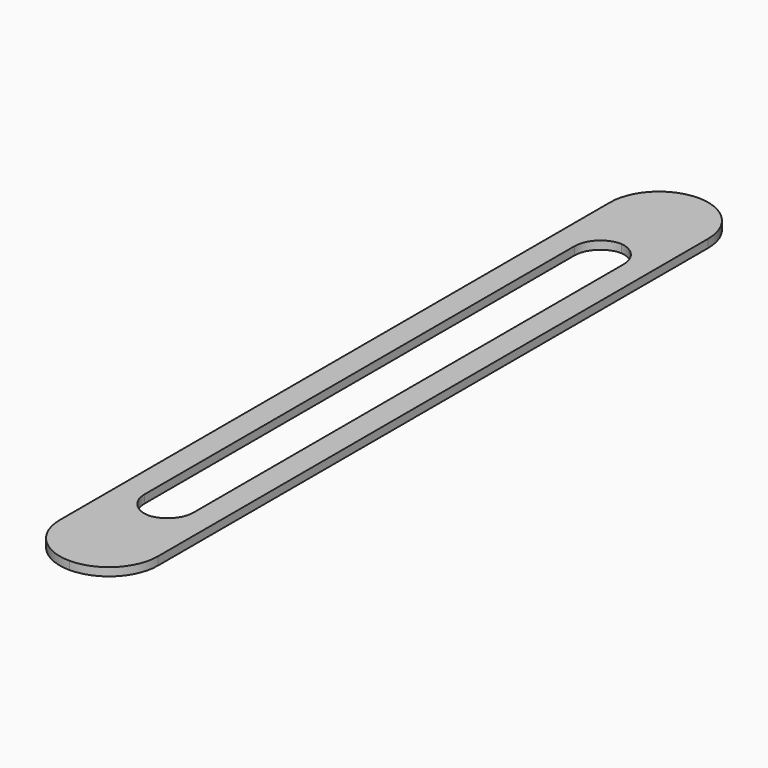
from build123d import *

# Parameters (mm, degrees)
F0_W        = 19.05
F0_H        = 152.4
F1_DEPTH    = 1.5875
F2_R        = 9.52499
F4_W        = 9.525
F4_H        = 114.3
F5_DEPTH    = 25.4
F6_T1_DEPTH = 1.5875
F7_T1_DEPTH = 1.5875


# Not quite as in the source:
# - a fillet or chamfer that OpenCascade refuses, or shapes differently, is made with other operations: its cross-section is extruded or revolved along the edge and cut away or added
# - a fillet or chamfer is up to 0.001 mm smaller than in the source, because OpenCascade refuses the exact size


with BuildPart() as f1:
    # F0 (on Top) → F1 (new body)
    with BuildSketch(Plane.XY):
        with Locations((-58.0996136427, 28.9993500233)):
            Rectangle(F0_W, F0_H)
    extrude(amount=-F1_DEPTH)

    # F2 (radius 9.525 in the source; OpenCascade refuses exactly that, so slightly less here)
    f2_edges = [f1.edges().sort_by_distance(p)[0] for p in [
        (-48.574614, -47.20065, -0.79375),
        (-67.624614, -47.20065, -0.79375),
        (-48.574614, 105.19935, -0.79375),
        (-67.624614, 105.19935, -0.79375),
    ]]
    fillet(f2_edges, radius=F2_R)

    # F4 (on offset) → F5 (cut)
    with BuildSketch(Plane.XY):
        with Locations((-58.0996136427, 28.9993500233)):
            Rectangle(F4_W, F4_H)
    extrude(amount=-F5_DEPTH, mode=Mode.SUBTRACT)

    # F6: fillet of radius 5.08 on 3 edges, made by hand

    # F6_s2 → F6_t1 (join)
    with BuildSketch(Plane.XY.offset(-1.5875)):
        with BuildLine():
            ThreePointArc((-62.8621136427, -23.0706499767), (-61.3742160911, -26.6627524252), (-57.7821136427, -28.1506499767))
            Line((-57.7821136427, -28.1506499767), (-62.8621136427, -28.1506499767))
            Line((-62.8621136427, -28.1506499767), (-62.8621136427, -23.0706499767))
        make_face()
        with BuildLine():
            ThreePointArc((-57.7821136427, 86.1493500233), (-61.3742160911, 84.6614524717), (-62.8621136427, 81.0693500233))
            Line((-62.8621136427, 81.0693500233), (-62.8621136427, 86.1493500233))
            Line((-62.8621136427, 86.1493500233), (-57.7821136427, 86.1493500233))
        make_face()
        with BuildLine():
            ThreePointArc((-58.4171136427, -28.1506499767), (-54.8250111943, -26.6627524252), (-53.3371136427, -23.0706499767))
            Line((-53.3371136427, -23.0706499767), (-53.3371136427, -28.1506499767))
            Line((-53.3371136427, -28.1506499767), (-58.4171136427, -28.1506499767))
        make_face()
    extrude(amount=F6_T1_DEPTH)

    # F7: fillet of radius 5.08 on 1 edges, made by hand

    # F7_s2 → F7_t1 (join)
    with BuildSketch(Plane.XY.offset(-1.5875)):
        with BuildLine():
            ThreePointArc((-57.7821136427, 86.1493500233), (-54.6071136427, 84.4692979408), (-53.3371136427, 81.1091937757))
            Line((-53.3371136427, 81.1091937757), (-53.3371136427, 86.1493500233))
            Line((-53.3371136427, 86.1493500233), (-57.7821136427, 86.1493500233))
        make_face()
    extrude(amount=F7_T1_DEPTH)


solid = f1.part
